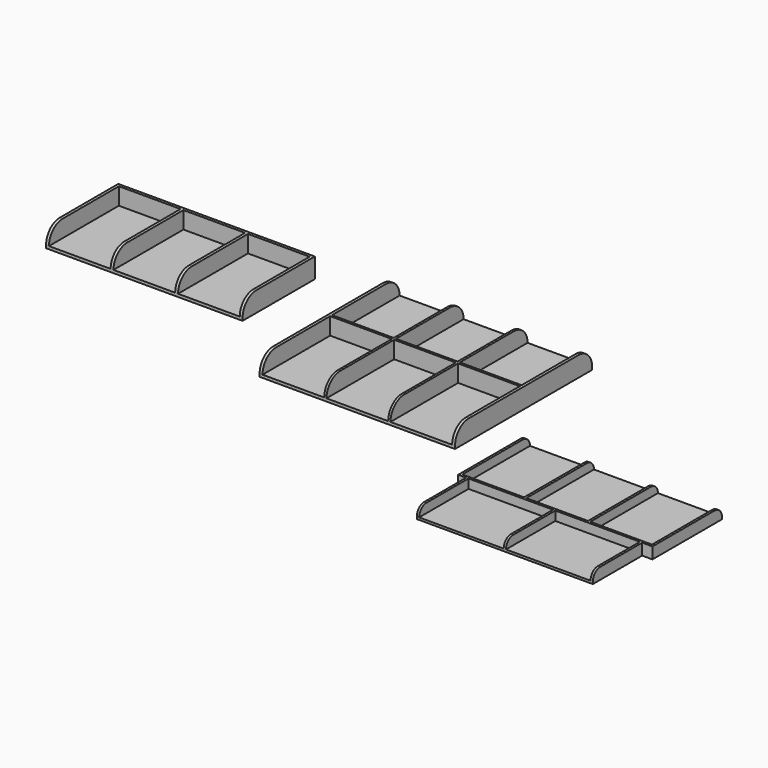
from build123d import *

# Parameters (mm, degrees)
F0_W      = 172
F0_H      = 79
F0_W_2    = 54
F0_H_2    = 74
F1_DEPTH  = 15
F2_W      = 172
F2_H      = 79
F2_W_2    = 54
F2_H_2    = 74
F3_DEPTH  = 2.5
F4_DEPTH  = 5
F5_R      = 15
F7_DEPTH  = 15
F6_W      = 54
F6_H      = 74
F8_DEPTH  = 2.5
F9_R      = 15
F10_W     = 2
F10_H     = 54
F11_DEPTH = 8
F10_W_2   = 74
F10_W_3   = 54
F10_H_2   = 74
F12_DEPTH = 2
F13_R     = 8
F14_ANGLE = 180


# Not quite as in the source:
# - a feature names something its author has since deleted; it is built from what else it names


with BuildPart() as f1:
    # F0 (on Top) → F1 (new body)
    with BuildSketch(Plane.XY):
        with Locations((-10.2776020169, 7.8872568756)):
            Rectangle(F0_W, F0_H)
        with Locations((-66.7776020169, 7.8872568756)):
            Rectangle(F0_W_2, F0_H_2, mode=Mode.SUBTRACT)
        with Locations((-10.2776020169, 7.8872568756)):
            Rectangle(F0_W_2, F0_H_2, mode=Mode.SUBTRACT)
        with Locations((46.2223979831, 7.8872568756)):
            Rectangle(F0_W_2, F0_H_2, mode=Mode.SUBTRACT)
    extrude(amount=F1_DEPTH)

    # F2 (on face) → F3 (join)
    with BuildSketch(Plane.XY.offset(15)):
        with Locations((-10.2776020169, 7.8872568756)):
            Rectangle(F2_W, F2_H)
        with Locations((-66.7776020169, 7.8872568756)):
            Rectangle(F2_W_2, F2_H_2, mode=Mode.SUBTRACT)
        with Locations((-10.2776020169, 7.8872568756)):
            Rectangle(F2_W_2, F2_H_2, mode=Mode.SUBTRACT)
        with Locations((46.2223979831, 7.8872568756)):
            Rectangle(F2_W_2, F2_H_2, mode=Mode.SUBTRACT)
        with Locations((-66.7776020169, 7.8872568756)):
            Rectangle(F2_W_2, F2_H_2)
        with Locations((-10.2776020169, 7.8872568756)):
            Rectangle(F2_W_2, F2_H_2)
        with Locations((46.2223979831, 7.8872568756)):
            Rectangle(F2_W_2, F2_H_2)
    extrude(amount=F3_DEPTH)

    # F4 (cut): faces of the model
    f4_faces = [f1.faces().sort_by_distance(p)[0] for p in [
        (-66.7776020169, -29.1127431244, 7.5),
        (-10.2776020169, -29.1127431244, 7.5),
        (46.2223979831, -29.1127431244, 7.5),
    ]]
    extrude(f4_faces, amount=-F4_DEPTH, mode=Mode.SUBTRACT)

    # F5
    f5_edges = [f1.edges().sort_by_distance(p)[0] for p in [
        (74.472398, -31.612743, 0),
        (17.972398, -31.612743, 0),
        (-38.527602, -31.612743, 0),
        (-95.027602, -31.612743, 0),
    ]]
    fillet(f5_edges, radius=F5_R)


with BuildPart() as f7:
    # F6 (on face) → F7 (new body)
    with BuildSketch(Plane(origin=(0, 0, 15), x_dir=(1, 0, 0), z_dir=(0, 0, -1))):
        Polygon((-159.6608362198, 13.0613436699), (-159.6608362198, -60.9386563301), (-157.1608362198, -60.8302913606), (-157.1608362198, 89.0613436699), (-159.6608362198, 89.0613436699), (-159.6608362198, 15.0613436699), (-213.6608362198, 15.0613436699), (-213.6608362198, 89.0613436699), (-215.6608362198, 89.0613436699), (-215.6608362198, 15.0613436699), (-269.6608362198, 15.0613436699), (-269.6608362198, 89.0613436699), (-271.6608362198, 89.0613436699), (-271.6608362198, 15.0613436699), (-325.6608362198, 15.0613436699), (-325.6608362198, 89.0613436699), (-328.1608362198, 89.0613436699), (-328.1608362198, -60.9386563301), (-325.6608362198, -60.9386563301), (-325.6608362198, 13.0613436699), (-271.6608362198, 13.0613436699), (-271.6608362198, -60.9386563301), (-269.6608362198, -60.9386563301), (-269.6608362198, 13.0613436699), (-215.6608362198, 13.0613436699), (-215.6608362198, -60.9386563301), (-213.6608362198, -60.9386563301), (-213.6608362198, 13.0613436699), align=None)
    extrude(amount=F7_DEPTH)

    # F6 (on face) → F8 (join)
    with BuildSketch(Plane(origin=(0, 0, 15), x_dir=(1, 0, 0), z_dir=(0, 0, -1))):
        with Locations((-186.6608362198, 52.0613436699)):
            Rectangle(F6_W, F6_H)
        with Locations((-242.6608362198, 52.0613436699)):
            Rectangle(F6_W, F6_H)
        with Locations((-298.6608362198, 52.0613436699)):
            Rectangle(F6_W, F6_H)
        with Locations((-298.6608362198, -23.9386563301)):
            Rectangle(F6_W, F6_H)
        with Locations((-242.6608362198, -23.9386563301)):
            Rectangle(F6_W, F6_H)
        with Locations((-186.6608362198, -23.9386563301)):
            Rectangle(F6_W, F6_H)
        Polygon((-159.6608362198, 13.0613436699), (-159.6608362198, -60.9386563301), (-157.1608362198, -60.8302913606), (-157.1608362198, 89.0613436699), (-159.6608362198, 89.0613436699), (-159.6608362198, 15.0613436699), (-213.6608362198, 15.0613436699), (-213.6608362198, 89.0613436699), (-215.6608362198, 89.0613436699), (-215.6608362198, 15.0613436699), (-269.6608362198, 15.0613436699), (-269.6608362198, 89.0613436699), (-271.6608362198, 89.0613436699), (-271.6608362198, 15.0613436699), (-325.6608362198, 15.0613436699), (-325.6608362198, 89.0613436699), (-328.1608362198, 89.0613436699), (-328.1608362198, -60.9386563301), (-325.6608362198, -60.9386563301), (-325.6608362198, 13.0613436699), (-271.6608362198, 13.0613436699), (-271.6608362198, -60.9386563301), (-269.6608362198, -60.9386563301), (-269.6608362198, 13.0613436699), (-215.6608362198, 13.0613436699), (-215.6608362198, -60.9386563301), (-213.6608362198, -60.9386563301), (-213.6608362198, 13.0613436699), align=None)
    extrude(amount=-F8_DEPTH)

    # F9
    f9_edges = [f7.edges().sort_by_distance(p)[0] for p in [
        (-158.410836, -89.061344, 0),
        (-214.660836, -89.061344, 0),
        (-158.410836, 60.884474, 0),
        (-214.660836, 60.938656, 0),
        (-270.660836, 60.938656, 0),
        (-326.910836, 60.938656, 0),
        (-326.910836, -89.061344, 0),
        (-270.660836, -89.061344, 0),
    ]]
    fillet(f9_edges, radius=F9_R)


with BuildPart() as f11:
    # F10 (on face) → F11 (new body)
    with BuildSketch(Plane(origin=(0, 0, 15), x_dir=(1, 0, 0), z_dir=(0, 0, -1))):
        Polygon((-368.2097992897, 131.1172200143), (-368.2097992897, 57.1172200143), (-366.2097992897, 57.1172200143), (-366.2097992897, 133.2441851207), (-373.2097992897, 133.1454344824), (-375.2097992897, 133.1172200143), (-449.2097992897, 133.1172200143), (-449.2097992897, 187.1172200143), (-451.2097992897, 187.1172200143), (-451.2097992897, 133.1172200143), (-525.2097992897, 133.1172200143), (-527.2097992897, 133.1172200143), (-536.2097992897, 133.1172200143), (-536.2097992897, 57.1172200143), (-534.2097992897, 57.1172200143), (-534.2097992897, 131.1172200143), (-480.2097992897, 131.1172200143), (-480.2097992897, 57.1172200143), (-478.2097992897, 57.1172200143), (-478.2097992897, 131.1172200143), (-424.2097992897, 131.1172200143), (-424.2097992897, 57.1172200143), (-422.2097992897, 57.1172200143), (-422.2097992897, 131.1172200143), align=None)
        Polygon((-375.2097992897, 133.1172200143), (-373.2097992897, 133.1454344824), (-373.2097992897, 187.1172200143), (-375.2097992897, 187.1172200143), align=None)
        with Locations((-526.2097992897, 160.1172200143)):
            Rectangle(F10_W, F10_H)
    extrude(amount=F11_DEPTH)

    # F10 (on face) → F12 (join)
    with BuildSketch(Plane(origin=(0, 0, 15), x_dir=(1, 0, 0), z_dir=(0, 0, -1))):
        Polygon((-375.2097992897, 133.1172200143), (-373.2097992897, 133.1454344824), (-373.2097992897, 187.1172200143), (-375.2097992897, 187.1172200143), align=None)
        Polygon((-368.2097992897, 131.1172200143), (-368.2097992897, 57.1172200143), (-366.2097992897, 57.1172200143), (-366.2097992897, 133.2441851207), (-373.2097992897, 133.1454344824), (-375.2097992897, 133.1172200143), (-449.2097992897, 133.1172200143), (-449.2097992897, 187.1172200143), (-451.2097992897, 187.1172200143), (-451.2097992897, 133.1172200143), (-525.2097992897, 133.1172200143), (-527.2097992897, 133.1172200143), (-536.2097992897, 133.1172200143), (-536.2097992897, 57.1172200143), (-534.2097992897, 57.1172200143), (-534.2097992897, 131.1172200143), (-480.2097992897, 131.1172200143), (-480.2097992897, 57.1172200143), (-478.2097992897, 57.1172200143), (-478.2097992897, 131.1172200143), (-424.2097992897, 131.1172200143), (-424.2097992897, 57.1172200143), (-422.2097992897, 57.1172200143), (-422.2097992897, 131.1172200143), align=None)
        with Locations((-412.2097992897, 160.1172200143)):
            Rectangle(F10_W_2, F10_H)
        with Locations((-395.2097992897, 94.1172200143)):
            Rectangle(F10_W_3, F10_H_2)
        with Locations((-451.2097992897, 94.1172200143)):
            Rectangle(F10_W_3, F10_H_2)
        with Locations((-507.2097992897, 94.1172200143)):
            Rectangle(F10_W_3, F10_H_2)
        with Locations((-526.2097992897, 160.1172200143)):
            Rectangle(F10_W, F10_H)
        with Locations((-488.2097992897, 160.1172200143)):
            Rectangle(F10_W_2, F10_H)
    extrude(amount=-F12_DEPTH)

    # F13
    f13_edges = [f11.edges().sort_by_distance(p)[0] for p in [
        (-374.209799, -187.11722, 7),
        (-367.209799, -57.11722, 7),
        (-423.209799, -57.11722, 7),
        (-450.209799, -187.11722, 7),
        (-526.209799, -187.11722, 7),
        (-535.209799, -57.11722, 7),
        (-479.209799, -57.11722, 7),
    ]]
    fillet(f13_edges, radius=F13_R)


with BuildPart() as f11_1:
    # F14: moved
    add(f11.part.rotate(Axis((-328.1608362198, -14.0613436699, 17.5), (0, -1, 0)), F14_ANGLE))


with BuildPart() as f7_1:
    # F14: moved
    add(f7.part.rotate(Axis((-328.1608362198, -14.0613436699, 17.5), (0, -1, 0)), F14_ANGLE))


with BuildPart() as f1_1:
    # F14: moved
    add(f1.part.rotate(Axis((-328.1608362198, -14.0613436699, 17.5), (0, -1, 0)), F14_ANGLE))


solid = Compound([f11_1.part, f7_1.part, f1_1.part])
